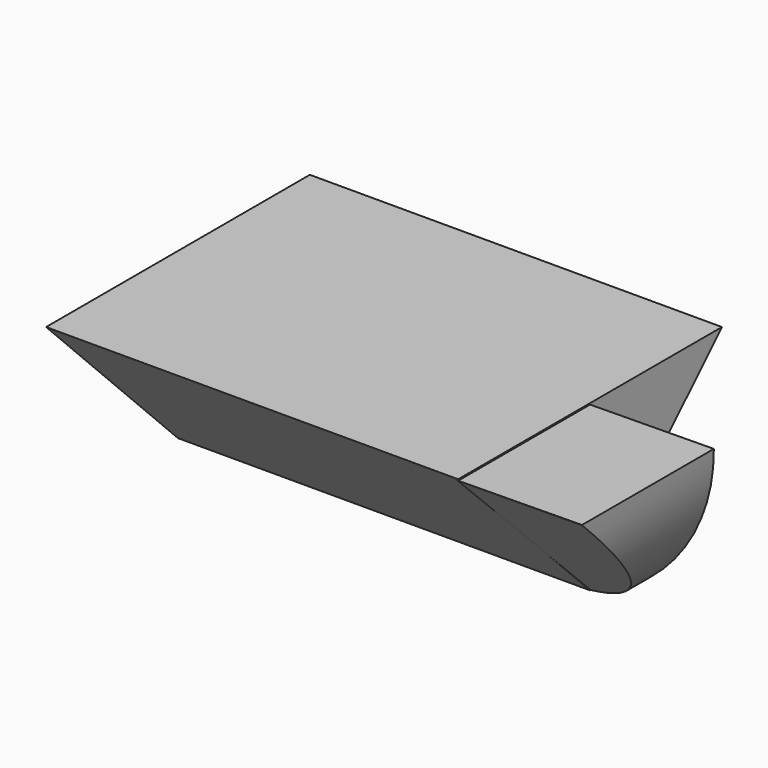
from build123d import *

# Parameters (mm, degrees)
F0_W        = 63.5
F0_H        = 76.2
F1_DEPTH    = 25.4
F2_T1_DEPTH = 259.462243683
F3_T1_DEPTH = 259.462243683
F5_DEPTH    = 25.4
F7_DEPTH    = 25.4


# Not quite as in the source:
# - a fillet or chamfer that OpenCascade refuses, or shapes differently, is made with other operations: its cross-section is extruded or revolved along the edge and cut away or added


with BuildPart() as f1:
    # F0 (on Top) → F1 (new body)
    with BuildSketch(Plane.XY):
        Rectangle(F0_W, F0_H)
    extrude(amount=-F1_DEPTH)

    # F2: chamfer of 38.1 on 1 edges, made by hand

    # F2_s2 → F2_t1 (cut)
    with BuildSketch(Plane.YZ.offset(-129.7311218415)):
        Polygon((38.1, 12.7), (0, -25.4), (38.1, -25.4), align=None)
    extrude(amount=F2_T1_DEPTH, mode=Mode.SUBTRACT)

    # F3: chamfer of 38.1 on 1 edges, made by hand

    # F3_s2 → F3_t1 (cut)
    with BuildSketch(Plane.YZ.offset(-129.7311218415)):
        Polygon((0, -25.4), (-38.1, 12.7), (-38.1, -25.4), align=None)
    extrude(amount=F3_T1_DEPTH, mode=Mode.SUBTRACT)

    # F4 (on Front) → F5 (join)
    with BuildSketch(Plane.XZ):
        with BuildLine():
            Line((31.6233746707, -0.1989824377), (31.8418294191, -25.3204219043))
            ThreePointArc((31.8418294191, -25.3204219043), (45.6070605547, -15.863879172), (50.8267469704, 0))
            Line((50.8267469704, 0), (31.6233746707, -0.1989824377))
        make_face()
    extrude(amount=F5_DEPTH)

    # F6 (on face) → F7 (cut)
    with BuildSketch(Plane(origin=(31.6192532968, 0, 0.274959404), x_dir=(0, -1, 0), z_dir=(-0.9999621924, 0, -0.0086956199))):
        Polygon((25.4, -0.473959761), (0, -25.5963490453), (25.4, -25.5963490453), align=None)
    extrude(amount=-F7_DEPTH, mode=Mode.SUBTRACT)


solid = f1.part
